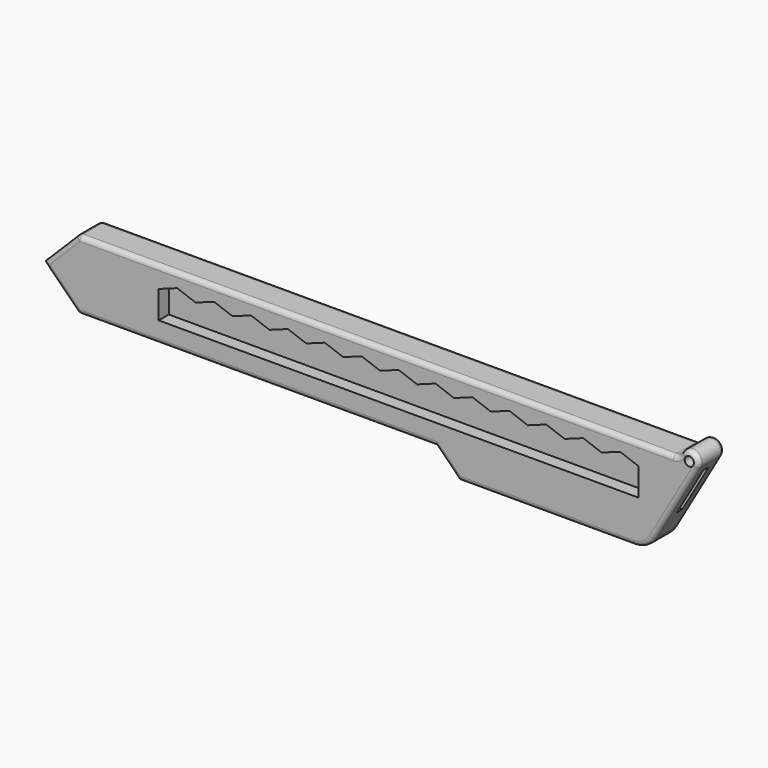
from build123d import *

# Parameters (mm, degrees)
F1_DEPTH     = 3.5
F3_DEPTH     = 3.501
F4_W         = 1.5
F4_H         = 10
F5_DEPTH     = 142.001
F6_R         = 1
F7_DEPTH     = 7.001
F8_R         = 2
F9_T1_DEPTH  = 131.5358983849
F9_T3_DEPTH  = 45.762395693
F9_T5_DEPTH  = 15.6066017178
F9_T7_DEPTH  = 15.6066017178
F9_T9_DEPTH  = 24.4393102292
F9_T14_DEPTH = 12.0710678119
F9_T19_DEPTH = 12.0710678119
F9_T24_DEPTH = 82.5
F9_T29_DEPTH = 82.5
F9_T32_ANGLE = 60
F9_T34_ANGLE = 180
F9_T36_ANGLE = 60
F9_T38_ANGLE = 180
F9_T43_DEPTH = 82.5
F9_T47_DEPTH = 12.0710678119
F9_T54_DEPTH = 82.5
F9_T58_DEPTH = 12.0710678119
F10_R        = 1
F11_T1_DEPTH = 6.9999999999
F11_T4_ANGLE = 60
F11_T6_ANGLE = 60


# Not quite as in the source:
# - a fillet or chamfer that OpenCascade refuses, or shapes differently, is made with other operations: its cross-section is extruded or revolved along the edge and cut away or added


with BuildPart() as f1:
    # F0 (on Front) → F1 (new body, symmetric)
    with BuildSketch(Plane.XZ):
        with BuildLine():
            Line((0, 0), (7.5, -7.5))
            Line((7.5, -7.5), (85, -7.5))
            Line((85, -7.5), (90, -12.5))
            Line((90, -12.5), (130.762395693, -12.5))
            Line((130.762395693, -12.5), (141.7320508076, 6.5))
            ThreePointArc((141.7320508076, 6.5), (140.5176380902, 9.4318516526), (138, 7.5))
            Line((138, 7.5), (7.5, 7.5))
            Line((7.5, 7.5), (0, 0))
        make_face()
    extrude(amount=F1_DEPTH, both=True)

    # F2 (on Front) → F3 (cut, through all)
    with BuildSketch(Plane.XZ):
        Polygon((29, 4.4558809371), (25, 3), (25, -3), (33, -3), (33, 3), align=None)
        Polygon((37, 4.4558809371), (33, 3), (33, -3), (41, -3), (49, -3), (57, -3), (65, -3), (73, -3), (81, -3), (89, -3), (97, -3), (105, -3), (113, -3), (121, -3), (129, -3), (129, 3), (125, 4.4558809371), (121, 3), (117, 4.4558809371), (113, 3), (109, 4.4558809371), (105, 3), (101, 4.4558809371), (97, 3), (93, 4.4558809371), (89, 3), (85, 4.4558809371), (81, 3), (77, 4.4558809371), (73, 3), (69, 4.4558809371), (65, 3), (61, 4.4558809371), (57, 3), (53, 4.4558809371), (49, 3), (45, 4.4558809371), (41, 3), align=None)
    extrude(amount=F3_DEPTH, mode=Mode.SUBTRACT)

    # F4 (on Right) → F5 (cut, through all)
    with BuildSketch(Plane.YZ):
        Rectangle(F4_W, F4_H)
    extrude(amount=F5_DEPTH, mode=Mode.SUBTRACT)

    # F6 (on face) → F7 (cut, through all)
    with BuildSketch(Plane.XZ.offset(3.5)):
        with Locations((140, 7.5)):
            Circle(F6_R)
    extrude(amount=-F7_DEPTH, mode=Mode.SUBTRACT)

    # F8
    f8_edges = [f1.edges().sort_by_distance(p)[0] for p in [
        (138, 0, 7.5),
    ]]
    fillet(f8_edges, radius=F8_R)

    # F9: fillet of radius 1 on 12 edges, made by hand

    # F9_s2 → F9_t1 (cut)
    with BuildSketch(Plane.YZ.offset(5)):
        with BuildLine():
            ThreePointArc((-2.5, 7.5), (-3.2071067812, 7.2071067812), (-3.5, 6.5))
            Line((-3.5, 6.5), (-3.5, 7.5))
            Line((-3.5, 7.5), (-2.5, 7.5))
        make_face()
        with BuildLine():
            ThreePointArc((2.5, 7.5), (3.2071067812, 7.2071067812), (3.5, 6.5))
            Line((3.5, 6.5), (3.5, 7.5))
            Line((3.5, 7.5), (2.5, 7.5))
        make_face()
    extrude(amount=F9_T1_DEPTH, mode=Mode.SUBTRACT)

    # F9_s4 → F9_t3 (cut)
    with BuildSketch(Plane.YZ.offset(87.5)):
        with BuildLine():
            ThreePointArc((-3.5, -11.5), (-3.2071067812, -12.2071067812), (-2.5, -12.5))
            Line((-2.5, -12.5), (-3.5, -12.5))
            Line((-3.5, -12.5), (-3.5, -11.5))
        make_face()
        with BuildLine():
            ThreePointArc((3.5, -11.5), (3.2071067812, -12.2071067812), (2.5, -12.5))
            Line((2.5, -12.5), (3.5, -12.5))
            Line((3.5, -12.5), (3.5, -11.5))
        make_face()
    extrude(amount=F9_T3_DEPTH, mode=Mode.SUBTRACT)

    # F9_s6 → F9_t5 (cut)
    with BuildSketch(Plane(origin=(-1.767766953, 0, 1.767766953), x_dir=(0, 1, 0), z_dir=(0.7071067812, 0, -0.7071067812))):
        with BuildLine():
            ThreePointArc((-3.5, 1), (-3.2071067812, 0.2928932188), (-2.5, 0))
            Line((-2.5, 0), (-3.5, 0))
            Line((-3.5, 0), (-3.5, 1))
        make_face()
        with BuildLine():
            ThreePointArc((3.5, 1), (3.2071067812, 0.2928932188), (2.5, 0))
            Line((2.5, 0), (3.5, 0))
            Line((3.5, 0), (3.5, 1))
        make_face()
    extrude(amount=F9_T5_DEPTH, mode=Mode.SUBTRACT)

    # F9_s8 → F9_t7 (cut)
    with BuildSketch(Plane(origin=(9.267766953, 0, 9.267766953), x_dir=(0, 1, 0), z_dir=(-0.7071067812, 0, -0.7071067812))):
        with BuildLine():
            ThreePointArc((-2.5, 0), (-3.2071067812, 0.2928932188), (-3.5, 1))
            Line((-3.5, 1), (-3.5, 0))
            Line((-3.5, 0), (-2.5, 0))
        make_face()
        with BuildLine():
            ThreePointArc((3.5, 1), (3.2071067812, 0.2928932188), (2.5, 0))
            Line((2.5, 0), (3.5, 0))
            Line((3.5, 0), (3.5, 1))
        make_face()
    extrude(amount=F9_T7_DEPTH, mode=Mode.SUBTRACT)

    # F9_s10 → F9_t9 (cut)
    with BuildSketch(Plane(origin=(26.0279401496, 0, 45.0817147554), x_dir=(0, 1, 0), z_dir=(0.5, 0, 0.8660254038))):
        with BuildLine():
            ThreePointArc((3.5, -118.4935565298), (3.2071067812, -119.200663311), (2.5, -119.4935565298))
            Line((2.5, -119.4935565298), (3.5, -119.4935565298))
            Line((3.5, -119.4935565298), (3.5, -118.4935565298))
        make_face()
        with BuildLine():
            ThreePointArc((-3.5, -118.4935565298), (-3.2071067812, -119.200663311), (-2.5, -119.4935565298))
            Line((-2.5, -119.4935565298), (-3.5, -119.4935565298))
            Line((-3.5, -119.4935565298), (-3.5, -118.4935565298))
        make_face()
    extrude(amount=F9_T9_DEPTH, mode=Mode.SUBTRACT)


with BuildPart() as f9_tool12:
    # F9_s13 → F9_t14 (new body)
    with BuildSketch(Plane(origin=(44.482233047, 0, -44.482233047), x_dir=(0, 1, 0), z_dir=(0.7071067812, 0, -0.7071067812))):
        with BuildLine():
            ThreePointArc((-3.5, 55.800775542), (-3.2071067812, 55.0936687608), (-2.5, 54.800775542))
            Line((-2.5, 54.800775542), (-3.5, 54.800775542))
            Line((-3.5, 54.800775542), (-3.5, 55.800775542))
        make_face()
    extrude(amount=F9_T14_DEPTH)

    split(bisect_by=Plane.XY.offset(-7.5), keep=Keep.BOTTOM)


with BuildPart() as f1_1:
    add(f1.part)

    # F9_t11: cut F9_tool12
    add(f9_tool12.part, mode=Mode.SUBTRACT)


with BuildPart() as f9_tool17:
    # F9_s18 → F9_t19 (new body)
    with BuildSketch(Plane(origin=(44.482233047, 0, -44.482233047), x_dir=(0, 1, 0), z_dir=(0.7071067812, 0, -0.7071067812))):
        with BuildLine():
            ThreePointArc((3.5, 55.800775542), (3.2071067812, 55.0936687608), (2.5, 54.800775542))
            Line((2.5, 54.800775542), (3.5, 54.800775542))
            Line((3.5, 54.800775542), (3.5, 55.800775542))
        make_face()
    extrude(amount=F9_T19_DEPTH)

    split(bisect_by=Plane.XY.offset(-7.5), keep=Keep.BOTTOM)


with BuildPart() as f1_2:
    add(f1_1.part)

    # F9_t16: cut F9_tool17
    add(f9_tool17.part, mode=Mode.SUBTRACT)


with BuildPart() as f9_tool22:
    # F9_s23 → F9_t24 (new body)
    with BuildSketch(Plane.YZ.offset(5)):
        with BuildLine():
            ThreePointArc((-3.5, -6.5), (-3.2071067812, -7.2071067812), (-2.5, -7.5))
            Line((-2.5, -7.5), (-3.5, -7.5))
            Line((-3.5, -7.5), (-3.5, -6.5))
        make_face()
    extrude(amount=F9_T24_DEPTH)

    split(bisect_by=Plane(origin=(38.75, 0, 38.75), x_dir=(0, 1, 0), z_dir=(-0.7071067812, 0, -0.7071067812)), keep=Keep.TOP)


with BuildPart() as f1_3:
    add(f1_2.part)

    # F9_t21: cut F9_tool22
    add(f9_tool22.part, mode=Mode.SUBTRACT)


with BuildPart() as f9_tool27:
    # F9_s28 → F9_t29 (new body)
    with BuildSketch(Plane.YZ.offset(5)):
        with BuildLine():
            ThreePointArc((3.5, -6.5), (3.2071067812, -7.2071067812), (2.5, -7.5))
            Line((2.5, -7.5), (3.5, -7.5))
            Line((3.5, -7.5), (3.5, -6.5))
        make_face()
    extrude(amount=F9_T29_DEPTH)

    split(bisect_by=Plane(origin=(38.75, 0, 38.75), x_dir=(0, 1, 0), z_dir=(-0.7071067812, 0, -0.7071067812)), keep=Keep.TOP)


with BuildPart() as f1_4:
    add(f1_3.part)

    # F9_t26: cut F9_tool27
    add(f9_tool27.part, mode=Mode.SUBTRACT)

    # F9_s31 → F9_t32 (revolve, cut)
    with BuildSketch(Plane.YZ.offset(136.5358983849)):
        with BuildLine():
            ThreePointArc((3.5, 6.5), (3.2071067812, 7.2071067812), (2.5, 7.5))
            Line((2.5, 7.5), (3.5, 7.5))
            Line((3.5, 7.5), (3.5, 6.5))
        make_face()
    revolve(axis=Axis((136.5358983849, 3.5, 9.5), (0, -1, 0)), revolution_arc=F9_T32_ANGLE, mode=Mode.SUBTRACT)

    # F9_s33 → F9_t34 (revolve, cut)
    with BuildSketch(Plane(origin=(38.2475952642, 0, 66.2467782649), x_dir=(0, 1, 0), z_dir=(-0.5, 0, -0.8660254038))):
        with BuildLine():
            ThreePointArc((3.5, 118.4935565298), (3.2071067812, 119.200663311), (2.5, 119.4935565298))
            Line((2.5, 119.4935565298), (3.5, 119.4935565298))
            Line((3.5, 119.4935565298), (3.5, 118.4935565298))
        make_face()
    revolve(axis=Axis((140, 3.5, 7.5), (0, -1, 0)), revolution_arc=F9_T34_ANGLE, mode=Mode.SUBTRACT)

    # F9_s35 → F9_t36 (revolve, cut)
    with BuildSketch(Plane.YZ.offset(136.5358983849)):
        with BuildLine():
            ThreePointArc((-2.5, 7.5), (-3.2071067812, 7.2071067812), (-3.5, 6.5))
            Line((-3.5, 6.5), (-3.5, 7.5))
            Line((-3.5, 7.5), (-2.5, 7.5))
        make_face()
    revolve(axis=Axis((136.5358983849, -3.5, 9.5), (0, -1, 0)), revolution_arc=F9_T36_ANGLE, mode=Mode.SUBTRACT)

    # F9_s37 → F9_t38 (revolve, cut)
    with BuildSketch(Plane(origin=(38.2475952642, 0, 66.2467782649), x_dir=(0, 1, 0), z_dir=(-0.5, 0, -0.8660254038))):
        with BuildLine():
            ThreePointArc((-3.5, 118.4935565298), (-3.2071067812, 119.200663311), (-2.5, 119.4935565298))
            Line((-2.5, 119.4935565298), (-3.5, 119.4935565298))
            Line((-3.5, 119.4935565298), (-3.5, 118.4935565298))
        make_face()
    revolve(axis=Axis((140, -3.5, 7.5), (0, -1, 0)), revolution_arc=F9_T38_ANGLE, mode=Mode.SUBTRACT)


with BuildPart() as f9_tool41:
    # F9_s42 → F9_t43 (new body)
    with BuildSketch(Plane.YZ.offset(5)):
        with BuildLine():
            ThreePointArc((-3.5, -6.5), (-3.2071067812, -7.2071067812), (-2.5, -7.5))
            Line((-2.5, -7.5), (-3.5, -7.5))
            Line((-3.5, -7.5), (-3.5, -6.5))
        make_face()
    extrude(amount=F9_T43_DEPTH)

    split(bisect_by=Plane(origin=(38.75, 0, 38.75), x_dir=(0, 1, 0), z_dir=(0.7071067812, 0, 0.7071067812)), keep=Keep.TOP)


with BuildPart() as f9_tool45:
    # F9_s46 → F9_t47 (new body)
    with BuildSketch(Plane(origin=(44.482233047, 0, -44.482233047), x_dir=(0, 1, 0), z_dir=(0.7071067812, 0, -0.7071067812))):
        with BuildLine():
            ThreePointArc((-3.5, 55.800775542), (-3.2071067812, 55.0936687608), (-2.5, 54.800775542))
            Line((-2.5, 54.800775542), (-3.5, 54.800775542))
            Line((-3.5, 54.800775542), (-3.5, 55.800775542))
        make_face()
    extrude(amount=F9_T47_DEPTH)

    split(bisect_by=Plane.XY.offset(-7.5), keep=Keep.TOP)


with BuildPart() as f9_tool41_1:
    add(f9_tool41.part)

    # F9_t49: intersect F9_tool45
    add(f9_tool45.part, mode=Mode.INTERSECT)


with BuildPart() as f1_5:
    add(f1_4.part)

    # F9_t39: cut F9_tool41
    add(f9_tool41_1.part, mode=Mode.SUBTRACT)


with BuildPart() as f9_tool52:
    # F9_s53 → F9_t54 (new body)
    with BuildSketch(Plane.YZ.offset(5)):
        with BuildLine():
            ThreePointArc((3.5, -6.5), (3.2071067812, -7.2071067812), (2.5, -7.5))
            Line((2.5, -7.5), (3.5, -7.5))
            Line((3.5, -7.5), (3.5, -6.5))
        make_face()
    extrude(amount=F9_T54_DEPTH)

    split(bisect_by=Plane(origin=(38.75, 0, 38.75), x_dir=(0, 1, 0), z_dir=(0.7071067812, 0, 0.7071067812)), keep=Keep.TOP)


with BuildPart() as f9_tool56:
    # F9_s57 → F9_t58 (new body)
    with BuildSketch(Plane(origin=(44.482233047, 0, -44.482233047), x_dir=(0, 1, 0), z_dir=(0.7071067812, 0, -0.7071067812))):
        with BuildLine():
            ThreePointArc((3.5, 55.800775542), (3.2071067812, 55.0936687608), (2.5, 54.800775542))
            Line((2.5, 54.800775542), (3.5, 54.800775542))
            Line((3.5, 54.800775542), (3.5, 55.800775542))
        make_face()
    extrude(amount=F9_T58_DEPTH)

    split(bisect_by=Plane.XY.offset(-7.5), keep=Keep.TOP)


with BuildPart() as f9_tool52_1:
    add(f9_tool52.part)

    # F9_t60: intersect F9_tool56
    add(f9_tool56.part, mode=Mode.INTERSECT)


with BuildPart() as f1_6:
    add(f1_5.part)

    # F9_t50: cut F9_tool52
    add(f9_tool52_1.part, mode=Mode.SUBTRACT)

    # F10
    f10_edges = [f1_6.edges().sort_by_distance(p)[0] for p in [
        (7.5, 0, 7.5),
        (7.5, 0, -7.5),
    ]]
    fillet(f10_edges, radius=F10_R)

    # F11: fillet of radius 5 on 1 edges, made by hand

    # F11_s2 → F11_t1 (cut)
    with BuildSketch(Plane.XZ.offset(-3.5)):
        with BuildLine():
            ThreePointArc((132.2057713659, -10), (130.375644347, -11.8301270189), (127.875644347, -12.5))
            Line((127.875644347, -12.5), (130.762395693, -12.5))
            Line((130.762395693, -12.5), (132.2057713659, -10))
        make_face()
    extrude(amount=F11_T1_DEPTH, mode=Mode.SUBTRACT)

    # F11_s3 → F11_t4 (revolve, cut)
    with BuildSketch(Plane(origin=(28.7213158226, 0, 49.7467782649), x_dir=(0, 1, 0), z_dir=(0.5, 0, 0.8660254038))):
        with BuildLine():
            ThreePointArc((3.5, -118.4935565299), (3.2071067812, -119.200663311), (2.5, -119.4935565298))
            Line((2.5, -119.4935565298), (3.5, -119.4935565298))
            Line((3.5, -119.4935565298), (3.5, -118.4935565299))
        make_face()
    revolve(axis=Axis((127.875644347, 3.5, -7.5), (0, 1, 0)), revolution_arc=F11_T4_ANGLE, mode=Mode.SUBTRACT)

    # F11_s5 → F11_t6 (revolve, cut)
    with BuildSketch(Plane.YZ.offset(127.875644347)):
        with BuildLine():
            ThreePointArc((-3.5, -11.5), (-3.2071067812, -12.2071067812), (-2.5, -12.5))
            Line((-2.5, -12.5), (-3.5, -12.5))
            Line((-3.5, -12.5), (-3.5, -11.5))
        make_face()
    revolve(axis=Axis((127.875644347, -3.5, -7.5), (0, -1, 0)), revolution_arc=F11_T6_ANGLE, mode=Mode.SUBTRACT)


solid = f1_6.part
